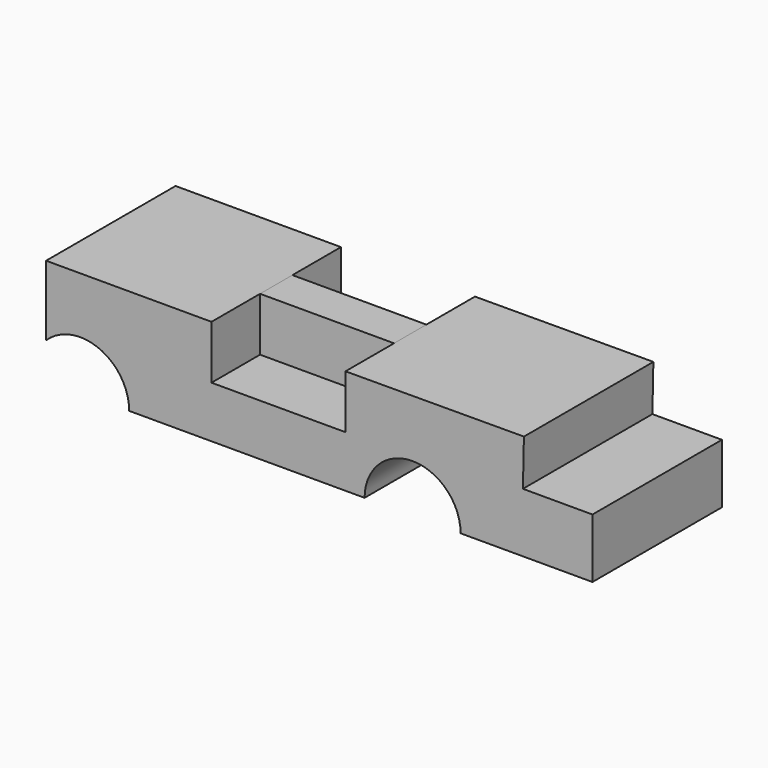
from build123d import *

# Parameters (mm, degrees)
F0_W     = 21.0292201075
F0_H     = 8.4116881791
F1_DEPTH = 3.175
F2_DEPTH = 12.7
F3_DEPTH = 12.7
F4_DEPTH = 12.7
F5_DEPTH = 3.175


# Not quite as in the source:
# - a length typed as a fraction of an inch, garbled in the dataset ("3 / 203.2 mm" for 3/8 in), is restored
# - the program builds the solid bodies; features that only make, move or delete a surface that nothing else refers to are left out


with BuildPart() as f1:
    # F0 (on Front) → F1 (new body, symmetric)
    with BuildSketch(Plane.XZ):
        with Locations((5.5916309617, -2.2130799996)):
            Rectangle(F0_W, F0_H)
        with BuildLine():
            Line((16.1062410154, -6.4189240892), (-4.9229790921, -6.4189240892))
            Line((-4.9229790921, -6.4189240892), (-4.9229790921, 1.9927640899))
            Line((-4.9229790921, 1.9927640899), (-22.6225737488, 1.9927640899))
            Line((-22.6225737488, 1.9927640899), (-30.8863221669, 1.9927640899))
            Line((-30.8863221669, 1.9927640899), (-30.8863221669, -9.0018421859))
            ThreePointArc((-30.8863221669, -9.0018421859), (-22.5331431268, -7.4335767863), (-17.836673191, -14.5172359101))
            Line((-17.836673191, -14.5172359101), (19.1034554321, -14.5172359101))
            ThreePointArc((19.1034554321, -14.5172359101), (26.6389876086, -6.9817037336), (34.174519785, -14.5172359101))
            Line((34.174519785, -14.5172359101), (48.1264702976, -14.5172359101))
            Line((48.1264702976, -14.5172359101), (54.8679456115, -14.5172359101))
            Line((54.8679456115, -14.5172359101), (54.8679456115, -5.1880707033))
            Line((54.8679456115, -5.1880707033), (43.9546283241, -5.1880707033))
            Line((43.9546283241, -5.1880707033), (44.1094860435, 2.0794970915))
            Line((44.1094860435, 2.0794970915), (16.1062410154, 1.9927640899))
            Line((16.1062410154, 1.9927640899), (16.1062410154, -6.4189240892))
        make_face()
    extrude(amount=F1_DEPTH, both=True)

    # F0 (on Front) → F2 (join, symmetric)
    with BuildSketch(Plane.XZ):
        with BuildLine():
            Line((16.1062410154, -6.4189240892), (-4.9229790921, -6.4189240892))
            Line((-4.9229790921, -6.4189240892), (-4.9229790921, 1.9927640899))
            Line((-4.9229790921, 1.9927640899), (-22.6225737488, 1.9927640899))
            Line((-22.6225737488, 1.9927640899), (-30.8863221669, 1.9927640899))
            Line((-30.8863221669, 1.9927640899), (-30.8863221669, -9.0018421859))
            ThreePointArc((-30.8863221669, -9.0018421859), (-22.5331431268, -7.4335767863), (-17.836673191, -14.5172359101))
            Line((-17.836673191, -14.5172359101), (19.1034554321, -14.5172359101))
            ThreePointArc((19.1034554321, -14.5172359101), (26.6389876086, -6.9817037336), (34.174519785, -14.5172359101))
            Line((34.174519785, -14.5172359101), (48.1264702976, -14.5172359101))
            Line((48.1264702976, -14.5172359101), (54.8679456115, -14.5172359101))
            Line((54.8679456115, -14.5172359101), (54.8679456115, -5.1880707033))
            Line((54.8679456115, -5.1880707033), (43.9546283241, -5.1880707033))
            Line((43.9546283241, -5.1880707033), (44.1094860435, 2.0794970915))
            Line((44.1094860435, 2.0794970915), (16.1062410154, 1.9927640899))
            Line((16.1062410154, 1.9927640899), (16.1062410154, -6.4189240892))
        make_face()
    extrude(amount=F2_DEPTH, both=True)

    # F0 (on Front) → F3 (join, symmetric)
    with BuildSketch(Plane.XZ):
        with BuildLine():
            Line((16.1062410154, -6.4189240892), (-4.9229790921, -6.4189240892))
            Line((-4.9229790921, -6.4189240892), (-4.9229790921, 1.9927640899))
            Line((-4.9229790921, 1.9927640899), (-22.6225737488, 1.9927640899))
            Line((-22.6225737488, 1.9927640899), (-30.8863221669, 1.9927640899))
            Line((-30.8863221669, 1.9927640899), (-30.8863221669, -9.0018421859))
            ThreePointArc((-30.8863221669, -9.0018421859), (-22.5331431268, -7.4335767863), (-17.836673191, -14.5172359101))
            Line((-17.836673191, -14.5172359101), (19.1034554321, -14.5172359101))
            ThreePointArc((19.1034554321, -14.5172359101), (26.6389876086, -6.9817037336), (34.174519785, -14.5172359101))
            Line((34.174519785, -14.5172359101), (48.1264702976, -14.5172359101))
            Line((48.1264702976, -14.5172359101), (54.8679456115, -14.5172359101))
            Line((54.8679456115, -14.5172359101), (54.8679456115, -5.1880707033))
            Line((54.8679456115, -5.1880707033), (43.9546283241, -5.1880707033))
            Line((43.9546283241, -5.1880707033), (44.1094860435, 2.0794970915))
            Line((44.1094860435, 2.0794970915), (16.1062410154, 1.9927640899))
            Line((16.1062410154, 1.9927640899), (16.1062410154, -6.4189240892))
        make_face()
    extrude(amount=F3_DEPTH, both=True)

    # F0 (on Front) → F4 (join, symmetric)
    with BuildSketch(Plane.XZ):
        with BuildLine():
            Line((16.1062410154, -6.4189240892), (-4.9229790921, -6.4189240892))
            Line((-4.9229790921, -6.4189240892), (-4.9229790921, 1.9927640899))
            Line((-4.9229790921, 1.9927640899), (-22.6225737488, 1.9927640899))
            Line((-22.6225737488, 1.9927640899), (-30.8863221669, 1.9927640899))
            Line((-30.8863221669, 1.9927640899), (-30.8863221669, -9.0018421859))
            ThreePointArc((-30.8863221669, -9.0018421859), (-22.5331431268, -7.4335767863), (-17.836673191, -14.5172359101))
            Line((-17.836673191, -14.5172359101), (19.1034554321, -14.5172359101))
            ThreePointArc((19.1034554321, -14.5172359101), (26.6389876086, -6.9817037336), (34.174519785, -14.5172359101))
            Line((34.174519785, -14.5172359101), (48.1264702976, -14.5172359101))
            Line((48.1264702976, -14.5172359101), (54.8679456115, -14.5172359101))
            Line((54.8679456115, -14.5172359101), (54.8679456115, -5.1880707033))
            Line((54.8679456115, -5.1880707033), (43.9546283241, -5.1880707033))
            Line((43.9546283241, -5.1880707033), (44.1094860435, 2.0794970915))
            Line((44.1094860435, 2.0794970915), (16.1062410154, 1.9927640899))
            Line((16.1062410154, 1.9927640899), (16.1062410154, -6.4189240892))
        make_face()
    extrude(amount=F4_DEPTH, both=True)


with BuildPart() as f5:
    # F0 (on Front) → F5 (new body, symmetric)
    with BuildSketch(Plane.XZ):
        with Locations((5.5916309617, -2.2130799996)):
            Rectangle(F0_W, F0_H)
    extrude(amount=F5_DEPTH, both=True)


solid = Compound([f1.part, f5.part])
